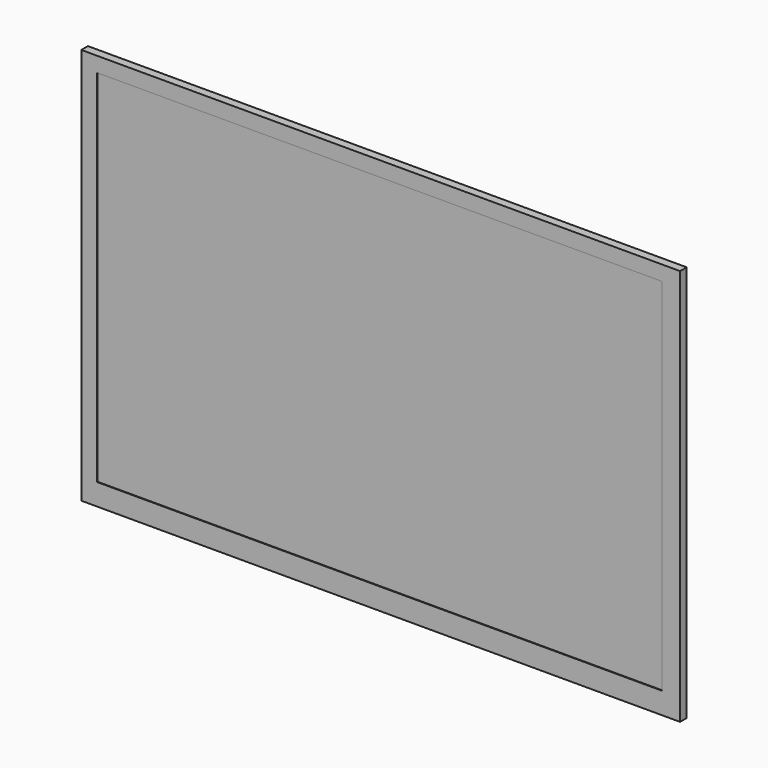
from build123d import *

# Parameters (mm, degrees)
F0_W     = 229.108
F0_H     = 151.8412
F1_DEPTH = 3.175
F2_W     = 216.154
F2_H     = 137.8712
F3_DEPTH = 0.254
F4_W     = 44.7675
F4_H     = 27.94
F5_DEPTH = 2.54
F7_DEPTH = 3.81
F8_R     = 3.80999


# Not quite as in the source:
# - a fillet or chamfer is up to 0.001 mm smaller than in the source, because OpenCascade refuses the exact size


with BuildPart() as f1:
    # F0 (on Front) → F1 (new body)
    with BuildSketch(Plane.XZ):
        with Locations((114.554, 75.9206)):
            Rectangle(F0_W, F0_H)
    extrude(amount=F1_DEPTH)

    # F2 (on face) → F3 (cut)
    with BuildSketch(Plane.XZ.offset(3.175)):
        with Locations((114.046, 77.1906)):
            Rectangle(F2_W, F2_H)
    extrude(amount=-F3_DEPTH, mode=Mode.SUBTRACT)

    # F4 (on face) → F5 (join)
    with BuildSketch(Plane(origin=(0, 0, 0), x_dir=(-1, 0, 0), z_dir=(0, 1, 0))):
        with Locations((-191.16675, 16.51)):
            Rectangle(F4_W, F4_H)
    extrude(amount=F5_DEPTH)

    # F6 (on face) → F7 (join)
    with BuildSketch(Plane(origin=(0, 2.54, 0), x_dir=(-1, 0, 0), z_dir=(0, 1, 0))):
        Polygon((-210.21675, 30.48), (-210.21675, 24.13), (-172.11675, 24.13), (-172.11675, 30.48), (-191.16675, 49.53), align=None)
    extrude(amount=F7_DEPTH)

    # F8 (radius 3.81 in the source; OpenCascade refuses exactly that, so slightly less here)
    f8_edges = [f1.edges().sort_by_distance(p)[0] for p in [
        (200.69175, 6.35, 40.005),
        (181.64175, 6.35, 40.005),
    ]]
    fillet(f8_edges, radius=F8_R)


solid = f1.part
